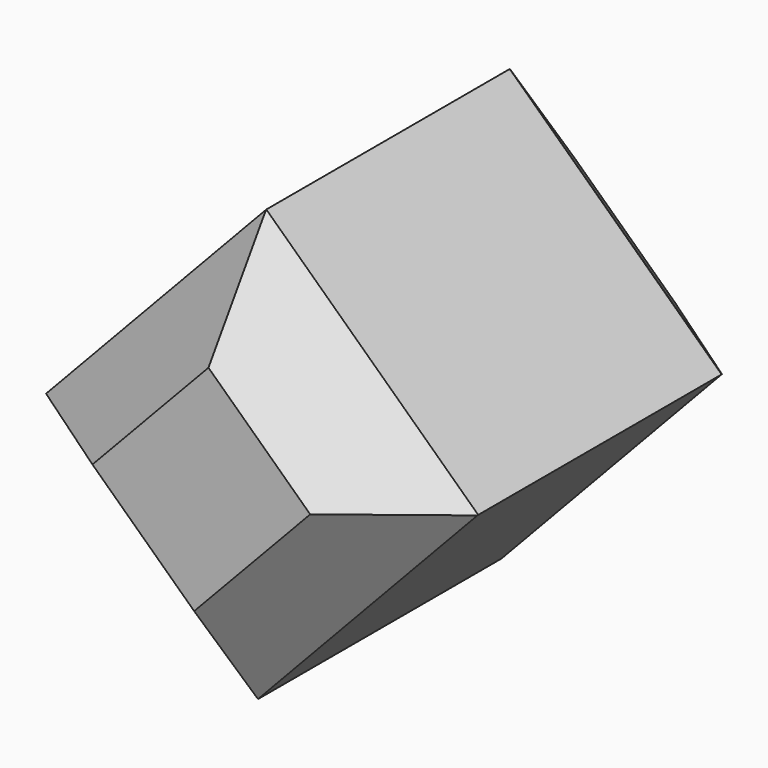
from build123d import *

# Parameters (mm, degrees)
F0_R      = 23.1993727041
F1_DEPTH  = 12.7
F2_R      = 23.1993727041
F3_DEPTH  = 12.7
F6_DEPTH  = 6.35
F7_DEPTH  = 6.35
F8_SIZE   = 6.34999
F9_SIZE   = 6.34999
F10_DEPTH = 25.4
F11_DEPTH = 127


# Not quite as in the source:
# - a fillet or chamfer is up to 0.001 mm smaller than in the source, because OpenCascade refuses the exact size


with BuildPart() as f1:
    # F0 (on Front) → F1 (new body)
    with BuildSketch(Plane.XZ):
        with Locations((-16.9251933694, -16.9251933694)):
            Circle(F0_R)
    extrude(amount=F1_DEPTH)

    # F2 (on face) → F3 (join)
    with BuildSketch(Plane(origin=(0, 0, 0), x_dir=(-1, 0, 0), z_dir=(0, 1, 0))):
        with Locations((16.9251933694, -16.9251933694)):
            Circle(F2_R)
    extrude(amount=F3_DEPTH)

    # F4 (on face) → F6 (join)
    with BuildSketch(Plane(origin=(0, 12.7, 0), x_dir=(-1, 0, 0), z_dir=(0, 1, 0))):
        Polygon((34.987336153, -18.3641740003), (16.5690030176, 1.1906780042), (-1.1369494142, -15.4862127385), (17.2813837212, -35.041064743), align=None)
    extrude(amount=F6_DEPTH)

    # F5 (on face) → F7 (join)
    with BuildSketch(Plane.XZ.offset(12.7)):
        Polygon((1.1413726115, -15.5428544637), (-16.5892601531, 1.1910649658), (-34.9917593503, -18.3075322751), (-17.2611265857, -35.0414517045), align=None)
    extrude(amount=F7_DEPTH)

    # F8 (size 6.35 in the source; OpenCascade refuses exactly that, so slightly less here)
    f8_edges = [f1.edges().sort_by_distance(p)[0] for p in [
        (-8.072217, 19.05, -25.263639),
        (-26.13436, 19.05, -26.702619),
        (-25.77817, 19.05, -8.586748),
        (-7.716027, 19.05, -7.147767),
    ]]
    chamfer(f8_edges, length=F8_SIZE)

    # F9 (size 6.35 in the source; OpenCascade refuses exactly that, so slightly less here)
    f9_edges = [f1.edges().sort_by_distance(p)[0] for p in [
        (-8.059877, -19.05, -25.292153),
        (-7.723944, -19.05, -7.175895),
        (-25.79051, -19.05, -8.558234),
        (-26.126443, -19.05, -26.674492),
    ]]
    chamfer(f9_edges, length=F9_SIZE)

    # F10 (cut): faces of the model
    f10_faces = [f1.faces().sort_by_distance(p)[0] for p in [
        (-39.4683887232, -12.7, -16.9251933694),
        (-39.4683887232, -12.7, -16.9251933694),
        (-39.4683887232, -12.7, -16.9251933694),
        (-39.4683887232, -12.7, -16.9251933694),
    ]]
    extrude(f10_faces, amount=-F10_DEPTH, mode=Mode.SUBTRACT)

    # F11 (cut): faces of the model
    f11_faces = [f1.faces().sort_by_distance(p)[0] for p in [
        (-6.6175325, 12.7, -23.7415572289),
        (-27.2328542388, 12.7, -10.1088295099),
    ]]
    extrude(f11_faces, amount=-F11_DEPTH, mode=Mode.SUBTRACT)


solid = f1.part
